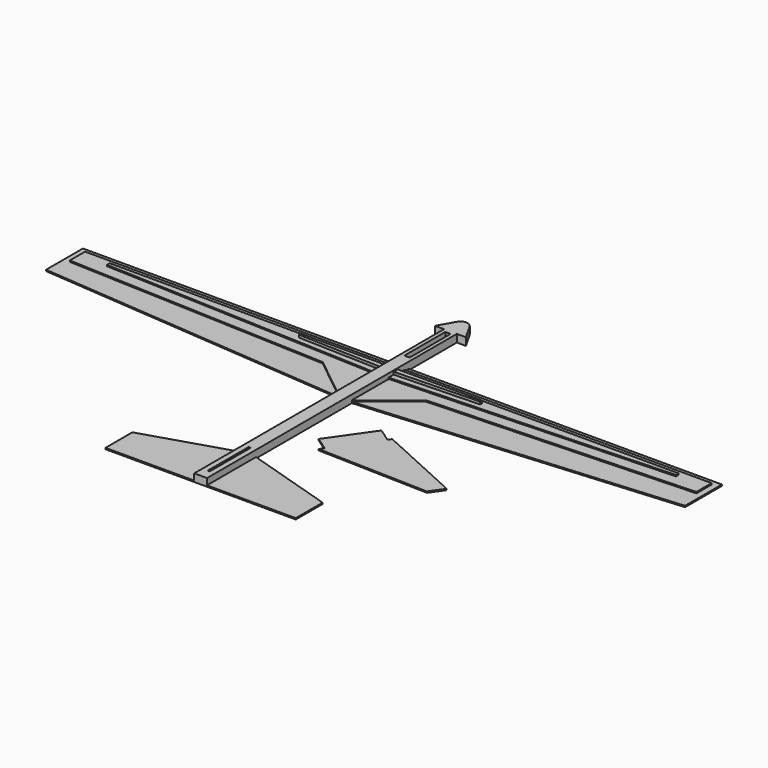
from build123d import *

# Parameters (mm, degrees)
F1_DEPTH = 0.5
F2_DEPTH = 3
F4_DEPTH = 0.5
F5_DEPTH = 0.5
F7_DEPTH = 0.5
F9_DEPTH = 1


# Not quite as in the source:
# - a feature names something its author has since deleted; it is built from what else it names


with BuildPart() as f1:
    # F0 (on Top) → F1 (new body)
    with BuildSketch(Plane.XY):
        Polygon((-2.5, -19.3782690912), (-2.5, 8.4829014608), (-125, 8.4829014608), (-125, 0), (-125, -9.5409080386), align=None)
        Polygon((-2.5, -90.2088385105), (-2.5, -66.2574071428), (-37.2240561792, -77.0772191324), (-37.2240561792, -90.2088385105), align=None)
        Polygon((37.2240561792, -77.0772191324), (2.5, -66.2574071428), (2.5, -90.2088385105), (37.2240561792, -90.2088385105), align=None)
        Polygon((125, 8.4829014608), (2.5, 8.4829014608), (2.5, -19.3782690912), (125, -9.5409080386), (125, 0), align=None)
        Polygon((2.5, 38.2264746347), (0, 38.2264746347), (-2.5, 38.2264746347), (-2.5, 31.9558866322), (-2.5, 8.4829014608), (-2.5, -19.3782690912), (-2.5, -66.2574071428), (-2.5, -90.2088385105), (0, -90.2088385105), (2.5, -90.2088385105), (2.5, -66.2574071428), (2.5, -19.3782690912), (2.5, 8.4829014608), (2.5, 31.9558866322), align=None)
        Polygon((-0.4, -66.2574071428), (0, -66.2574071428), (0.4, -66.2574071428), (0.4, -86.2574071428), (0, -86.2574071428), (-0.4, -86.2574071428), align=None, mode=Mode.SUBTRACT)
        Polygon((-1.05, 30.741930455), (0, 30.741930455), (1.05, 30.741930455), (1.05, 10.741930455), (0, 10.741930455), (-1.05, 10.741930455), align=None, mode=Mode.SUBTRACT)
    extrude(amount=F1_DEPTH)

    # F0 (on Top) → F2 (join)
    with BuildSketch(Plane.XY):
        Polygon((2.5, 38.2264746347), (0, 38.2264746347), (-2.5, 38.2264746347), (-2.5, 31.9558866322), (-2.5, 8.4829014608), (-2.5, -19.3782690912), (-2.5, -66.2574071428), (-2.5, -90.2088385105), (0, -90.2088385105), (2.5, -90.2088385105), (2.5, -66.2574071428), (2.5, -19.3782690912), (2.5, 8.4829014608), (2.5, 31.9558866322), align=None)
        Polygon((-0.4, -66.2574071428), (0, -66.2574071428), (0.4, -66.2574071428), (0.4, -86.2574071428), (0, -86.2574071428), (-0.4, -86.2574071428), align=None, mode=Mode.SUBTRACT)
        Polygon((-1.05, 30.741930455), (0, 30.741930455), (1.05, 30.741930455), (1.05, 10.741930455), (0, 10.741930455), (-1.05, 10.741930455), align=None, mode=Mode.SUBTRACT)
        Polygon((-2.5, 31.9558866322), (-2.5, 38.2264746347), (-6.0318950564, 31.9558866322), align=None)
        Polygon((6.0318950564, 31.9558866322), (2.5, 38.2264746347), (2.5, 31.9558866322), align=None)
        with BuildLine():
            Line((-2.5, 38.2264746347), (0, 38.2264746347))
            Line((0, 38.2264746347), (2.5, 38.2264746347))
            ThreePointArc((2.5, 38.2264746347), (0, 39.6876408194), (-2.5, 38.2264746347))
        make_face()
    extrude(amount=F2_DEPTH)

    # F3 (on face) → F4 (join)
    with BuildSketch(Plane.XY.offset(0.5)):
        Polygon((-2.5, -5.9316507274), (-2.5, 6.4829014608), (-122.5709915161, 6.4829014608), (-122.5709915161, -0.9700714727), (-20.2113245095, -5.1997825289), align=None)
        Polygon((122.5709915161, 6.4829014608), (0, 6.4829014608), (0, -6.034955847), (20.2113245095, -5.1997825289), (122.5709915161, -0.9700714727), align=None)
        Polygon((-2.5, -19.3782690912), (-2.5, -5.9316507274), (-20.2113245095, -5.1997825289), align=None)
        Polygon((20.2113245095, -5.1997825289), (0, -6.034955847), (0, -19.3782690912), (2.5, -19.3782690912), align=None)
    extrude(amount=F4_DEPTH)

    # F6 (on face) → F7 (join)
    with BuildSketch(Plane.XY.offset(1)):
        Polygon((111.3073602319, 4.4760769233), (0, 4.4760769233), (-111.3073602319, 4.4760769233), (-111.3073602319, 3.1342721807), (0, -1.4651758829), (111.3073602319, 3.1342721807), align=None)
    extrude(amount=F7_DEPTH)

    # F8 (on face) → F9 (join)
    with BuildSketch(Plane.XY.offset(1.5)):
        Polygon((-2.5, 1.0846625931), (-2.5, 3.1001814641), (-35.4501530528, 3.1001814641), (-35.4501530528, 2.1533293184), align=None)
        Polygon((35.4501530528, 3.1001814641), (0, 3.1001814641), (-2.5, 3.1001814641), (-2.5, 1.0846625931), (0, 1.0035805171), (35.4501530528, 2.1533293184), align=None)
    extrude(amount=F9_DEPTH)


with BuildPart() as f5:
    # F0 (on Top) → F5 (new body)
    with BuildSketch(Plane.XY):
        Polygon((15.2214128825, -48.6049928758), (14.1352575937, -50.1561833865), (57.4773901376, -51.3879905945), (61.0969997942, -46.2186522782), (27.5726027584, -30.9656656737), (26.6929416095, -32.22195199), (21.4564287133, -28.5553061862), (9.9848999862, -44.9383470719), align=None)
    extrude(amount=F5_DEPTH)


solid = Compound([f1.part, f5.part])
